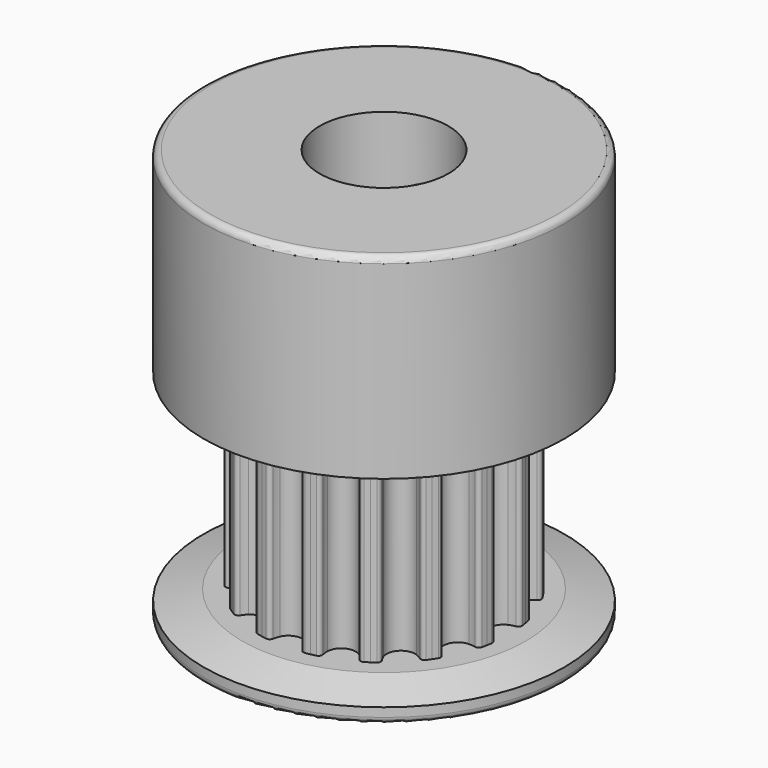
from build123d import *

# Parameters (mm, degrees)
F3_DEPTH    = 3.5
F4_COUNT    = 16
F5_R        = 7
F6_DEPTH    = 1
F7_R        = 7
F8_DEPTH    = 1
F9_R        = 7
F10_DEPTH   = 7
F11_R       = 2.5
F12_DEPTH   = 16.001
F13_R       = 1.75
F14_DEPTH   = 7.001
F15_R       = 1.75
F16_DEPTH   = 7.0010001
F17_SIZE2   = 0.4019237886
F17_SIZE    = 1.5
F17_2_SIZE2 = 0.4019237886
F17_2_SIZE  = 1.5
F18_R       = 0.25


# Not quite as in the source:
# - a feature names something its author has since deleted; it is built from what else it names


with BuildPart() as f3:
    # F2 (on Top) → F3 (new body, symmetric)
    with BuildSketch(Plane.XY):
        with BuildLine():
            ThreePointArc((0.5070084573, 4.4150779199), (0.3022651059, 4.1753692078), (0, 4.0858375803))
            ThreePointArc((0, 4.0858375803), (-0.3022651059, 4.1753692078), (-0.5070084573, 4.4150779199))
            ThreePointArc((-0.5070084573, 4.4150779199), (-0.5510572691, 4.5336764254), (-0.5797791871, 4.6568874426))
            ThreePointArc((-0.5797791871, 4.6568874426), (-0.6400054613, 4.7538203484), (-0.7510040389, 4.7803252181))
            ThreePointArc((-0.7510040389, 4.7803252181), (-0.8476929444, 4.7641298187), (-0.9440339094, 4.7459789544))
            Line((-0.9440339094, 4.7459789544), (0, 0))
            Line((0, 0), (0.9440339094, 4.7459789544))
            ThreePointArc((0.9440339094, 4.7459789544), (0.8476929444, 4.7641298187), (0.7510040389, 4.7803252181))
            ThreePointArc((0.7510040389, 4.7803252181), (0.6400054613, 4.7538203484), (0.5797791871, 4.6568874426))
            ThreePointArc((0.5797791871, 4.6568874426), (0.5510572691, 4.5336764254), (0.5070084573, 4.4150779199))
        make_face()
    extrude(amount=F3_DEPTH, both=True)

    # F4: F3 ×16 about axis
    f4_axis = Axis((0, 0, 0), (0, 0, -1))


with BuildPart() as f3_1:
    add(f3.part)
    for i in range(1, F4_COUNT):
        add(f3.part.rotate(f4_axis, i * 360 / F4_COUNT))

    # F5 (on face) → F6 (join)
    with BuildSketch(Plane(origin=(0, 0, -3.5), x_dir=(1, 0, 0), z_dir=(0, 0, -1))):
        Circle(F5_R)
    extrude(amount=F6_DEPTH)

    # F7 (on face) → F8 (join)
    with BuildSketch(Plane.XY.offset(3.5)):
        Circle(F7_R)
    extrude(amount=F8_DEPTH)

    # F9 (on face) → F10 (join)
    with BuildSketch(Plane.XY.offset(4.5)):
        Circle(F9_R)
    extrude(amount=F10_DEPTH)

    # F11 (on face) → F12 (cut, through all)
    with BuildSketch(Plane.XY.offset(11.5)):
        Circle(F11_R)
    extrude(amount=-F12_DEPTH, mode=Mode.SUBTRACT)

    # F13 (on Front) → F14 (cut, through all)
    with BuildSketch(Plane.XZ):
        with Locations((0, 7.5)):
            Circle(F13_R)
    extrude(amount=-F14_DEPTH, mode=Mode.SUBTRACT)

    # F15 (on Right) → F16 (cut, through all)
    with BuildSketch(Plane.YZ):
        with Locations((0, 7.5)):
            Circle(F15_R)
    extrude(amount=-F16_DEPTH, mode=Mode.SUBTRACT)

    # F17
    f17_edges = [f3_1.edges().sort_by_distance(p)[0] for p in [
        (-7, 0, -3.5),
    ]]
    f17_side = f3_1.faces().sort_by_distance((-6.80201, 0, -3.5))[0]
    chamfer(f17_edges, length=F17_SIZE, length2=F17_SIZE2, reference=f17_side)

    # F17#2
    f17_2_edges = [f3_1.edges().sort_by_distance(p)[0] for p in [
        (-7, 0, 3.5),
    ]]
    f17_2_side = f3_1.faces().sort_by_distance((-6.80201, 0, 3.5))[0]
    chamfer(f17_2_edges, length=F17_2_SIZE, length2=F17_2_SIZE2, reference=f17_2_side)

    # F18
    f18_edges = [f3_1.edges().sort_by_distance(p)[0] for p in [
        (-7, 0, 11.5),
        (-7, 0, -4.5),
    ]]
    fillet(f18_edges, radius=F18_R)


solid = f3_1.part
